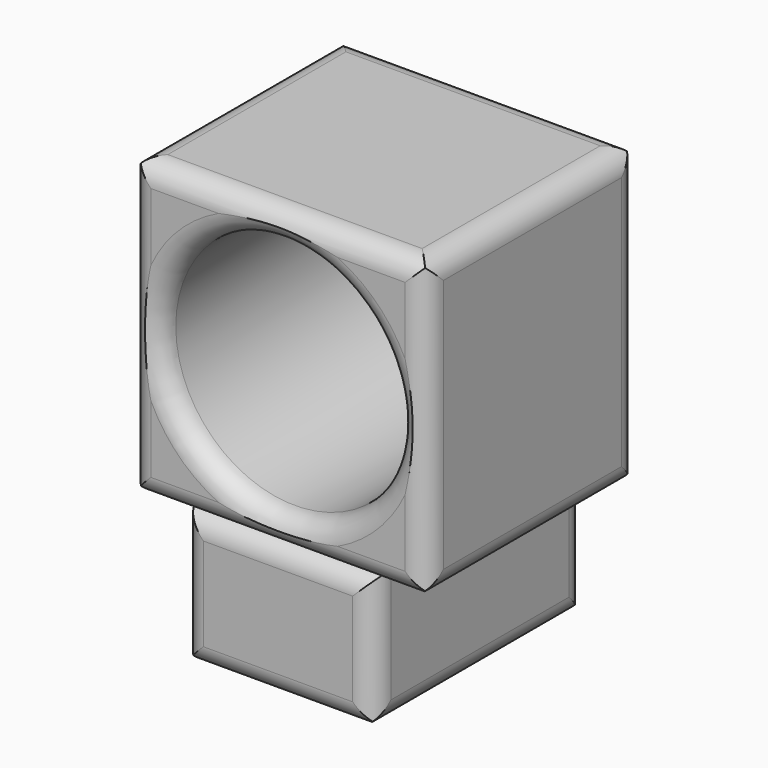
from build123d import *

# Parameters (mm, degrees)
F0_W          = 71.12
F0_H          = 71.12
F1_DEPTH      = 63.5
F2_R          = 28.575
F4_DEPTH      = 60.96
F5_T1_DEPTH   = 96.52
F5_T3_DEPTH   = 96.52
F6_R          = 5.08
F7_T1_DEPTH   = 78.74
F8_T1_DEPTH   = 78.74
F9_T1_DEPTH   = 78.74
F3_W          = 45.9716618061
F3_H          = 32.0539326784
F10_DEPTH     = 63.5
F11_T1_DEPTH  = 69.2741215893
F11_T3_DEPTH  = 71.3716618061
F11_T8_DEPTH  = 44.7539326784
F11_S9_R      = 5.0800000001
F11_T10_DEPTH = 24
F11_T14_DEPTH = 44.7539326784
F11_S15_R     = 5.0800000001
F11_T16_DEPTH = 24
F12_T1_DEPTH  = 71.3716618061
F12_T3_DEPTH  = 83.82
F13_T1_DEPTH  = 69.2741215891
F13_T6_DEPTH  = 39.6739326784
F13_S7_R      = 5.08
F13_T8_DEPTH  = 22
F13_T12_DEPTH = 39.6739326784
F13_S13_R     = 5.08
F13_T14_DEPTH = 22


# Not quite as in the source:
# - a fillet or chamfer that OpenCascade refuses, or shapes differently, is made with other operations: its cross-section is extruded or revolved along the edge and cut away or added


with BuildPart() as f1:
    # F0 (on Front) → F1 (new body)
    with BuildSketch(Plane.XZ):
        Rectangle(F0_W, F0_H)
    extrude(amount=F1_DEPTH)

    # F2 (on face) → F4 (cut)
    with BuildSketch(Plane.XZ.offset(63.5)):
        Circle(F2_R)
    extrude(amount=-F4_DEPTH, mode=Mode.SUBTRACT)

    # F5: fillet of radius 5.08 on 5 edges, made by hand

    # F5_s2 → F5_t1 (cut)
    with BuildSketch(Plane.YZ.offset(-48.26)):
        with BuildLine():
            ThreePointArc((-58.42, 35.56), (-62.0121024484, 34.0721024484), (-63.5, 30.48))
            Line((-63.5, 30.48), (-63.5, 35.56))
            Line((-63.5, 35.56), (-58.42, 35.56))
        make_face()
        with BuildLine():
            ThreePointArc((-63.5, -30.48), (-62.0121024484, -34.0721024484), (-58.42, -35.56))
            Line((-58.42, -35.56), (-63.5, -35.56))
            Line((-63.5, -35.56), (-63.5, -30.48))
        make_face()
    extrude(amount=F5_T1_DEPTH, mode=Mode.SUBTRACT)

    # F5_s4 → F5_t3 (cut)
    with BuildSketch(Plane.XY.offset(-48.26)):
        with BuildLine():
            ThreePointArc((35.56, -58.42), (34.0721024484, -62.0121024484), (30.48, -63.5))
            Line((30.48, -63.5), (35.56, -63.5))
            Line((35.56, -63.5), (35.56, -58.42))
        make_face()
        with BuildLine():
            ThreePointArc((-35.56, -58.42), (-34.0721024484, -62.0121024484), (-30.48, -63.5))
            Line((-30.48, -63.5), (-35.56, -63.5))
            Line((-35.56, -63.5), (-35.56, -58.42))
        make_face()
    extrude(amount=F5_T3_DEPTH, mode=Mode.SUBTRACT)

    # F5_s5 → F5_t6 (revolve, cut)
    with BuildSketch(Plane.XY):
        with BuildLine():
            ThreePointArc((33.655, -63.5), (30.0628975516, -62.0121024484), (28.575, -58.42))
            Line((28.575, -58.42), (28.575, -63.5))
            Line((28.575, -63.5), (33.655, -63.5))
        make_face()
    revolve(axis=Axis((0, -63.5, 0), (0, -1, 0)), mode=Mode.SUBTRACT)

    # F6
    f6_edges = [f1.edges().sort_by_distance(p)[0] for p in [
        (0, 0, 35.56),
        (-35.56, 0, 0),
        (0, 0, -35.56),
        (35.56, 0, 0),
    ]]
    fillet(f6_edges, radius=F6_R)

    # F7: fillet of radius 5.08 on 4 edges, made by hand

    # F7_s2 → F7_t1 (cut)
    with BuildSketch(Plane.XZ.offset(-7.62)):
        with BuildLine():
            ThreePointArc((-30.48, 35.56), (-34.0721024484, 34.0721024484), (-35.56, 30.48))
            Line((-35.56, 30.48), (-35.56, 35.56))
            Line((-35.56, 35.56), (-30.48, 35.56))
        make_face()
        with BuildLine():
            ThreePointArc((30.48, 35.56), (34.0721024484, 34.0721024484), (35.56, 30.48))
            Line((35.56, 30.48), (35.56, 35.56))
            Line((35.56, 35.56), (30.48, 35.56))
        make_face()
    extrude(amount=F7_T1_DEPTH, mode=Mode.SUBTRACT)

    # F8: fillet of radius 5.08 on 4 edges, made by hand

    # F8_s2 → F8_t1 (cut)
    with BuildSketch(Plane.XZ.offset(-7.62)):
        with BuildLine():
            ThreePointArc((35.56, -30.48), (34.0721024484, -34.0721024484), (30.48, -35.56))
            Line((30.48, -35.56), (35.56, -35.56))
            Line((35.56, -35.56), (35.56, -30.48))
        make_face()
    extrude(amount=F8_T1_DEPTH, mode=Mode.SUBTRACT)

    # F9: fillet of radius 5.08 on 4 edges, made by hand

    # F9_s2 → F9_t1 (cut)
    with BuildSketch(Plane.XZ.offset(-7.62)):
        with BuildLine():
            ThreePointArc((-35.56, -30.48), (-34.0721024484, -34.0721024484), (-30.48, -35.56))
            Line((-30.48, -35.56), (-35.56, -35.56))
            Line((-35.56, -35.56), (-35.56, -30.48))
        make_face()
    extrude(amount=F9_T1_DEPTH, mode=Mode.SUBTRACT)

    # F3 (on Front) → F10 (join)
    with BuildSketch(Plane.XZ):
        with Locations((0, -51.1674582958)):
            Rectangle(F3_W, F3_H)
    extrude(amount=F10_DEPTH)

    # F11: fillet of radius 5.08 on 4 edges, made by hand

    # F11_s2 → F11_t1 (cut)
    with BuildSketch(Plane.YZ.offset(-34.6370607946)):
        with BuildLine():
            ThreePointArc((-60.4414387753, -35.1404919566), (-62.6670759929, -37.0137369721), (-63.5, -39.8009839132))
            Line((-63.5, -39.8009839132), (-63.5, -35.1404919566))
            Line((-63.5, -35.1404919566), (-60.4414387753, -35.1404919566))
        make_face()
    extrude(amount=F11_T1_DEPTH, mode=Mode.SUBTRACT)

    # F11_s4 → F11_t3 (cut)
    with BuildSketch(Plane.YZ.offset(-35.6858309031)):
        with BuildLine():
            ThreePointArc((-63.5, -62.114424635), (-62.0121024484, -65.7065270835), (-58.42, -67.194424635))
            Line((-58.42, -67.194424635), (-63.5, -67.194424635))
            Line((-63.5, -67.194424635), (-63.5, -62.114424635))
        make_face()
    extrude(amount=F11_T3_DEPTH, mode=Mode.SUBTRACT)


with BuildPart() as f11_tool6:
    # F11_s7 → F11_t8 (new body)
    with BuildSketch(Plane.XY.offset(-35.1404919566)):
        with BuildLine():
            ThreePointArc((-22.9858309031, -58.42), (-21.4979333515, -62.0121024484), (-17.9058309031, -63.5))
            Line((-17.9058309031, -63.5), (-22.9858309031, -63.5))
            Line((-22.9858309031, -63.5), (-22.9858309031, -58.42))
        make_face()
    extrude(amount=-F11_T8_DEPTH)

    # F11_s9 → F11_t10 (cut, symmetric)
    with BuildSketch(Plane.YZ.offset(-20.4)):
        with Locations((-58.4199999999, -30.4799999999)):
            Circle(F11_S9_R)
    extrude(amount=F11_T10_DEPTH, both=True, mode=Mode.SUBTRACT)


with BuildPart() as f1_1:
    add(f1.part)

    # F11_t5: cut F11_tool6
    add(f11_tool6.part, mode=Mode.SUBTRACT)


with BuildPart() as f11_tool12:
    # F11_s13 → F11_t14 (new body)
    with BuildSketch(Plane.XY.offset(-79.894424635)):
        with BuildLine():
            ThreePointArc((22.9858309031, -58.42), (21.4979333515, -62.0121024484), (17.9058309031, -63.5))
            Line((17.9058309031, -63.5), (22.9858309031, -63.5))
            Line((22.9858309031, -63.5), (22.9858309031, -58.42))
        make_face()
    extrude(amount=F11_T14_DEPTH)

    # F11_s15 → F11_t16 (cut, symmetric)
    with BuildSketch(Plane.YZ.offset(20.4)):
        with Locations((-58.4199999999, -30.4799999999)):
            Circle(F11_S15_R)
    extrude(amount=F11_T16_DEPTH, both=True, mode=Mode.SUBTRACT)


with BuildPart() as f1_2:
    add(f1_1.part)

    # F11_t11: cut F11_tool12
    add(f11_tool12.part, mode=Mode.SUBTRACT)

    # F12: fillet of radius 5.08 on 4 edges, made by hand

    # F12_s2 → F12_t1 (cut)
    with BuildSketch(Plane.YZ.offset(-35.6858309031)):
        with BuildLine():
            ThreePointArc((0, -62.114424635), (-1.4878975516, -65.7065270835), (-5.08, -67.194424635))
            Line((-5.08, -67.194424635), (0, -67.194424635))
            Line((0, -67.194424635), (0, -62.114424635))
        make_face()
    extrude(amount=F12_T1_DEPTH, mode=Mode.SUBTRACT)

    # F12_s4 → F12_t3 (cut)
    with BuildSketch(Plane.XZ.offset(-12.7)):
        with BuildLine():
            ThreePointArc((22.9858309031, -62.114424635), (21.4979333515, -65.7065270835), (17.9058309031, -67.194424635))
            Line((17.9058309031, -67.194424635), (22.9858309031, -67.194424635))
            Line((22.9858309031, -67.194424635), (22.9858309031, -62.114424635))
        make_face()
        with BuildLine():
            ThreePointArc((-22.9858309031, -62.114424635), (-21.4979333515, -65.7065270835), (-17.9058309031, -67.194424635))
            Line((-17.9058309031, -67.194424635), (-22.9858309031, -67.194424635))
            Line((-22.9858309031, -67.194424635), (-22.9858309031, -62.114424635))
        make_face()
    extrude(amount=F12_T3_DEPTH, mode=Mode.SUBTRACT)

    # F13: fillet of radius 5.08 on 4 edges, made by hand

    # F13_s2 → F13_t1 (cut)
    with BuildSketch(Plane.YZ.offset(-34.6370607945)):
        with BuildLine():
            ThreePointArc((-3.0585612247, -35.1404919566), (-0.8329240071, -37.0137369721), (0, -39.8009839132))
            Line((0, -39.8009839132), (0, -35.1404919566))
            Line((0, -35.1404919566), (-3.0585612247, -35.1404919566))
        make_face()
    extrude(amount=F13_T1_DEPTH, mode=Mode.SUBTRACT)


with BuildPart() as f13_tool4:
    # F13_s5 → F13_t6 (new body)
    with BuildSketch(Plane.XY.offset(-74.814424635)):
        with BuildLine():
            ThreePointArc((22.9858309031, -5.08), (21.4979333515, -1.4878975516), (17.9058309031, 0))
            Line((17.9058309031, 0), (22.9858309031, 0))
            Line((22.9858309031, 0), (22.9858309031, -5.08))
        make_face()
    extrude(amount=F13_T6_DEPTH)

    # F13_s7 → F13_t8 (cut, symmetric)
    with BuildSketch(Plane.YZ.offset(20.4)):
        with Locations((-5.08, -30.48)):
            Circle(F13_S7_R)
    extrude(amount=F13_T8_DEPTH, both=True, mode=Mode.SUBTRACT)


with BuildPart() as f1_3:
    add(f1_2.part)

    # F13_t3: cut F13_tool4
    add(f13_tool4.part, mode=Mode.SUBTRACT)


with BuildPart() as f13_tool10:
    # F13_s11 → F13_t12 (new body)
    with BuildSketch(Plane.XY.offset(-35.1404919566)):
        with BuildLine():
            ThreePointArc((-22.9858309031, -5.08), (-21.4979333515, -1.4878975516), (-17.9058309031, 0))
            Line((-17.9058309031, 0), (-22.9858309031, 0))
            Line((-22.9858309031, 0), (-22.9858309031, -5.08))
        make_face()
    extrude(amount=-F13_T12_DEPTH)

    # F13_s13 → F13_t14 (cut, symmetric)
    with BuildSketch(Plane.YZ.offset(-20.4)):
        with Locations((-5.08, -30.48)):
            Circle(F13_S13_R)
    extrude(amount=F13_T14_DEPTH, both=True, mode=Mode.SUBTRACT)


with BuildPart() as f1_4:
    add(f1_3.part)

    # F13_t9: cut F13_tool10
    add(f13_tool10.part, mode=Mode.SUBTRACT)


solid = f1_4.part
